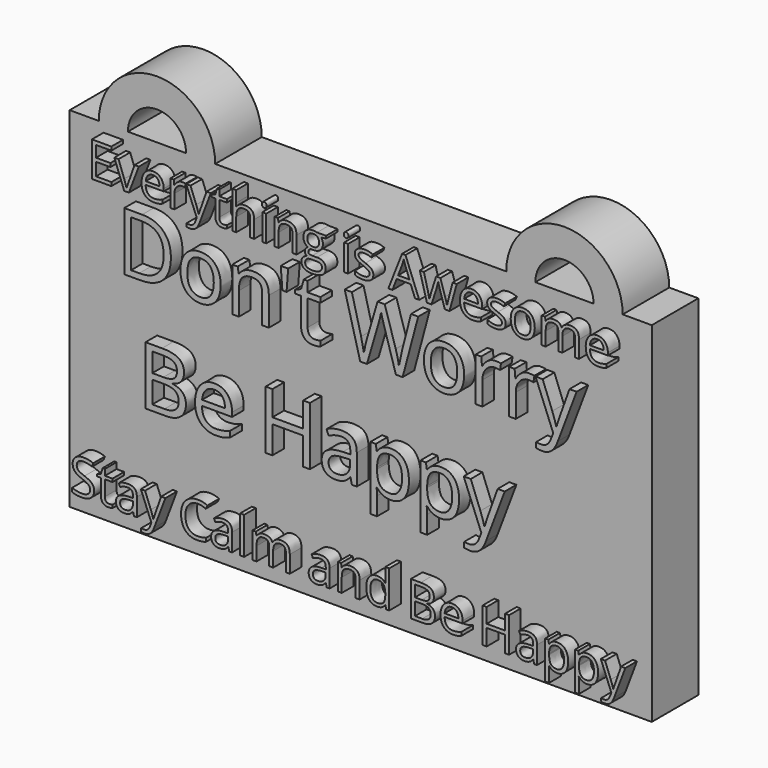
from build123d import *

# Parameters (mm, degrees)
F1_DEPTH       = 12.7
F2_TEXT_SIZE   = 17.8397212544
F2_TEXT_SIZE_2 = 10.6475990339
F2_TEXT_SIZE_3 = 10.6644896055
F3_DEPTH       = 3.175


# Not quite as in the source:
# - Text() gives the source's letters only with a copy of the font that has no kerning and outlines rounded to 1/6400 em; it was checked with that copy


with BuildPart() as f1:
    # F0 (on Front) → F1 (new body)
    with BuildSketch(Plane.XZ):
        with BuildLine():
            Line((-38.1, 38.1), (-31.75, 38.1))
            ThreePointArc((-31.75, 38.1), (-44.45, 50.8), (-57.15, 38.1))
            Line((-57.15, 38.1), (-50.8, 38.1))
            ThreePointArc((-50.8, 38.1), (-44.45, 44.45), (-38.1, 38.1))
        make_face()
        with BuildLine():
            Line((50.8, 38.1), (57.15, 38.1))
            ThreePointArc((57.15, 38.1), (44.45, 50.8), (31.75, 38.1))
            Line((31.75, 38.1), (38.1, 38.1))
            ThreePointArc((38.1, 38.1), (44.45, 44.45), (50.8, 38.1))
        make_face()
        Polygon((63.5, -38.1), (63.5, 38.1), (57.15, 38.1), (50.8, 38.1), (38.1, 38.1), (31.75, 38.1), (-31.75, 38.1), (-38.1, 38.1), (-50.8, 38.1), (-57.15, 38.1), (-63.5, 38.1), (-63.5, -38.1), align=None)
    extrude(amount=F1_DEPTH)

    # F2 (on face) → F3 (join)
    with BuildSketch(Plane.XZ.offset(12.7)):
        with Locations((-50.8, 12.5554006969)):
            Text("Don't Worry", F2_TEXT_SIZE, font='Open Sans', text_align=(TextAlign.LEFT, TextAlign.BOTTOM))
        with Locations((-46.1644599303, -11.7066202091)):
            Text('Be Happy', F2_TEXT_SIZE, font='Open Sans', text_align=(TextAlign.LEFT, TextAlign.BOTTOM))
        with Locations((-60.96, -33.2108706075)):
            Text('Stay Calm and Be Happy', F2_TEXT_SIZE_2, font='Open Sans', text_align=(TextAlign.LEFT, TextAlign.BOTTOM))
        with Locations((-57.15, 28.575)):
            Text('Everything is Awesome', F2_TEXT_SIZE_3, font='Open Sans', text_align=(TextAlign.LEFT, TextAlign.BOTTOM))
    extrude(amount=F3_DEPTH)


solid = f1.part
